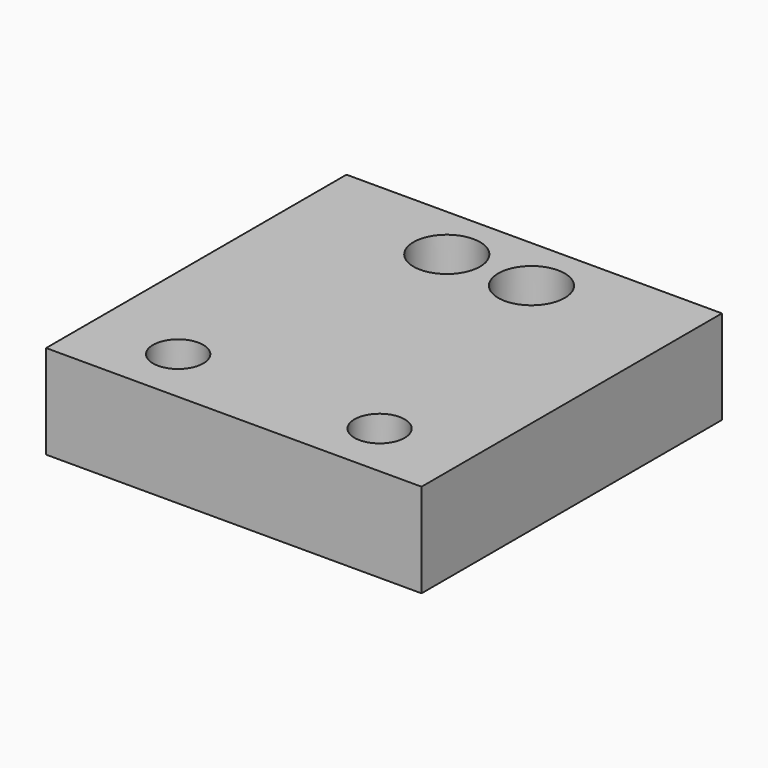
from build123d import *

# Parameters (mm, degrees)
F0_W     = 25.4
F0_H     = 25.4
F0_R     = 1.7
F0_R_2   = 0.75
F1_DEPTH = 6.35
F2_R     = 2.5
F3_DEPTH = 3.175
F4_R     = 2.25
F5_DEPTH = 3.75


# Not quite as in the source:
# - a feature names something its author has since deleted; it is built from what else it names


with BuildPart() as f1:
    # F0 (on Top) → F1 (new body)
    with BuildSketch(Plane.XY):
        Rectangle(F0_W, F0_H)
        with Locations((-6.8136113696, -8.89)):
            Circle(F0_R, mode=Mode.SUBTRACT)
        with Locations((6.8136113696, -8.89)):
            Circle(F0_R, mode=Mode.SUBTRACT)
        with Locations((-2.865, 8.89)):
            Circle(F0_R_2, mode=Mode.SUBTRACT)
        with Locations((2.865, 8.89)):
            Circle(F0_R_2, mode=Mode.SUBTRACT)
    extrude(amount=F1_DEPTH)

    # F2 (on Top) → F3 (cut)
    with BuildSketch(Plane.XY):
        with Locations((-6.8136113696, -8.89)):
            Circle(F2_R)
        with Locations((6.8136113696, -8.89)):
            Circle(F2_R)
    extrude(amount=F3_DEPTH, mode=Mode.SUBTRACT)

    # F4 (on face) → F5 (cut)
    with BuildSketch(Plane.XY.offset(6.35)):
        with Locations((-2.865, 8.89)):
            Circle(F4_R)
        with Locations((2.865, 8.89)):
            Circle(F4_R)
    extrude(amount=-F5_DEPTH, mode=Mode.SUBTRACT)


solid = f1.part
